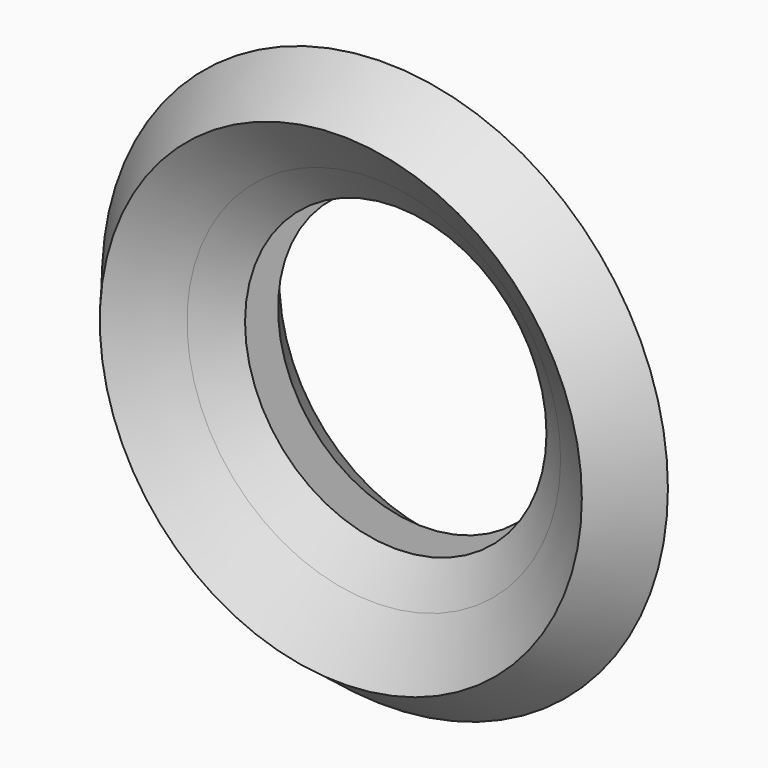
from build123d import *

# Parameters (mm, degrees)
F1_R     = 151.4348983765
F3_DEPTH = 25.4


# Not quite as in the source:
# - a feature of the source that left no trace in its solid (it failed there, or was rolled back) is left out


with BuildPart() as f2:
    # F0 (on Top) → F2 (revolve)
    with BuildSketch(Plane.XY):
        with BuildLine():
            Line((-14.491534441, -20.1198276415), (25.2444504306, -50.344484377))
            Line((25.2444504306, -50.344484377), (55.999001405, -9.9118540599))
            Line((55.999001405, -9.9118540599), (16.2630163267, 20.3128028329))
            ThreePointArc((16.2630163267, 20.3128028329), (23.6425286685, 11.3787127289), (26.2857406446, 0.0964878225))
            ThreePointArc((26.2857406446, 0.0964878225), (12.1679658867, -22.6603000349), (-14.491534441, -20.1198276415))
        make_face()
    revolve(axis=Axis((-151.4348983765, 0, 0), (0, -1, 0)))


with BuildPart() as f2b:
    # F0 (on Top) → F2, piece 2 (revolve)
    with BuildSketch(Plane.XY):
        with BuildLine():
            Line((-55.6208102037, 11.1646175717), (-14.491534441, -20.1198276415))
            ThreePointArc((-14.491534441, -20.1198276415), (-19.3305745926, 15.4737632063), (16.2630163267, 20.3128028329))
            Line((16.2630163267, 20.3128028329), (-24.8662592294, 51.5972478889))
            Line((-24.8662592294, 51.5972478889), (-55.6208102037, 11.1646175717))
        make_face()
    revolve(axis=Axis((-151.4348983765, 0, 0), (0, -1, 0)))

    # F1 (on Front) → F3 (cut)
    with BuildSketch(Plane.XZ):
        with Locations((-151.4348983765, 0)):
            Circle(F1_R)
    extrude(amount=-F3_DEPTH, mode=Mode.SUBTRACT)


solid = Compound([f2.part, f2b.part])
